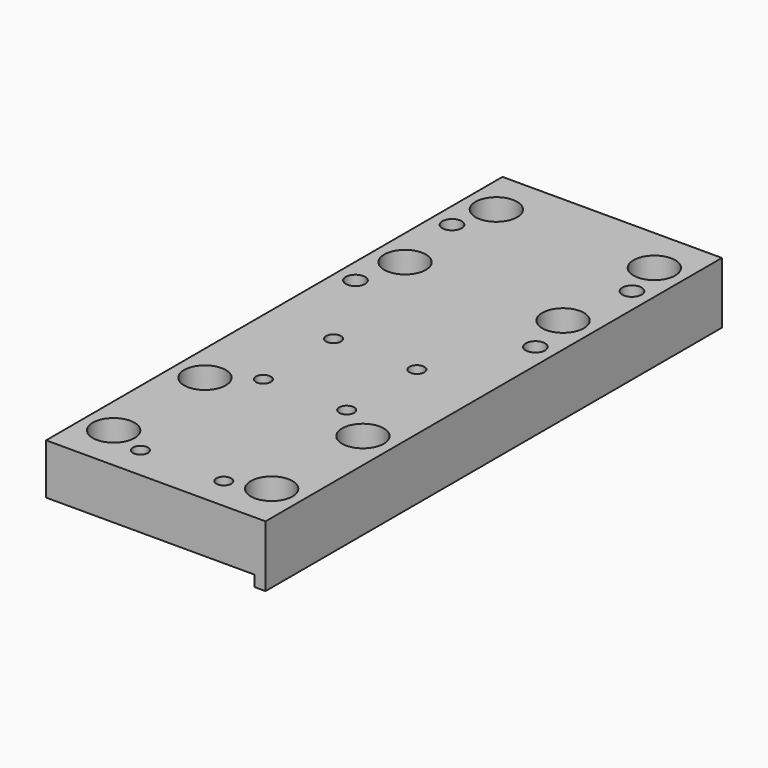
from build123d import *

# Parameters (mm, degrees)
F1_DEPTH = 130
F2_R     = 5.5
F3_DEPTH = 25
F2_R_2   = 9.5
F4_DEPTH = 13
F6_D     = 6.8
F7_D     = 8.8


# Not quite as in the source:
# - a pattern or mirror of a feature is missing from the dataset's text; its kind, count and spacing are read off the source's solid


with BuildPart() as f1:
    # F0 (on Front) → F1 (new body, symmetric)
    with BuildSketch(Plane.XZ):
        Polygon((-50, 23), (-50, 0), (45, 0), (45, -5), (50, -5), (50, 23), align=None)
    extrude(amount=F1_DEPTH, both=True)

    # F2 (on face) → F3 (cut)
    with BuildSketch(Plane.XY.offset(23)):
        with Locations((-36, -109)):
            Circle(F2_R)
        with Locations((36, -109)):
            Circle(F2_R)
        with Locations((-36, -57)):
            Circle(F2_R)
        with Locations((36, -57)):
            Circle(F2_R)
    f3 = extrude(amount=-F3_DEPTH, mode=Mode.SUBTRACT)

    # F3_copies: F3 across plane
    add(f3.mirror(Plane.ZX), mode=Mode.SUBTRACT)

    # F2 (on face) → F4 (cut)
    with BuildSketch(Plane.XY.offset(23)):
        with Locations((-36, -109)):
            Circle(F2_R_2)
        with Locations((-36, -109)):
            Circle(F2_R, mode=Mode.SUBTRACT)
        with Locations((36, -109)):
            Circle(F2_R_2)
        with Locations((36, -109)):
            Circle(F2_R, mode=Mode.SUBTRACT)
        with Locations((36, -109)):
            Circle(F2_R)
        with Locations((-36, -57)):
            Circle(F2_R_2)
        with Locations((-36, -57)):
            Circle(F2_R, mode=Mode.SUBTRACT)
        with Locations((36, -57)):
            Circle(F2_R_2)
        with Locations((36, -57)):
            Circle(F2_R, mode=Mode.SUBTRACT)
        with Locations((36, -57)):
            Circle(F2_R)
    f4 = extrude(amount=-F4_DEPTH, mode=Mode.SUBTRACT)

    # F4_copies: F4 across plane
    add(f4.mirror(Plane.ZX), mode=Mode.SUBTRACT)

    # F6 (through all)
    with Locations(Plane.XY.offset(23)):
        with Locations((-19, -115), (19, -115), (-19, -45), (19, -45), (19, -5), (-19, -5)):
            Hole(F6_D / 2)

    # F7 (through all)
    with Locations(Plane.XY.offset(23)):
        with Locations((-41, 35), (41, 35), (41, 90), (-41, 90)):
            Hole(F7_D / 2)


solid = f1.part
